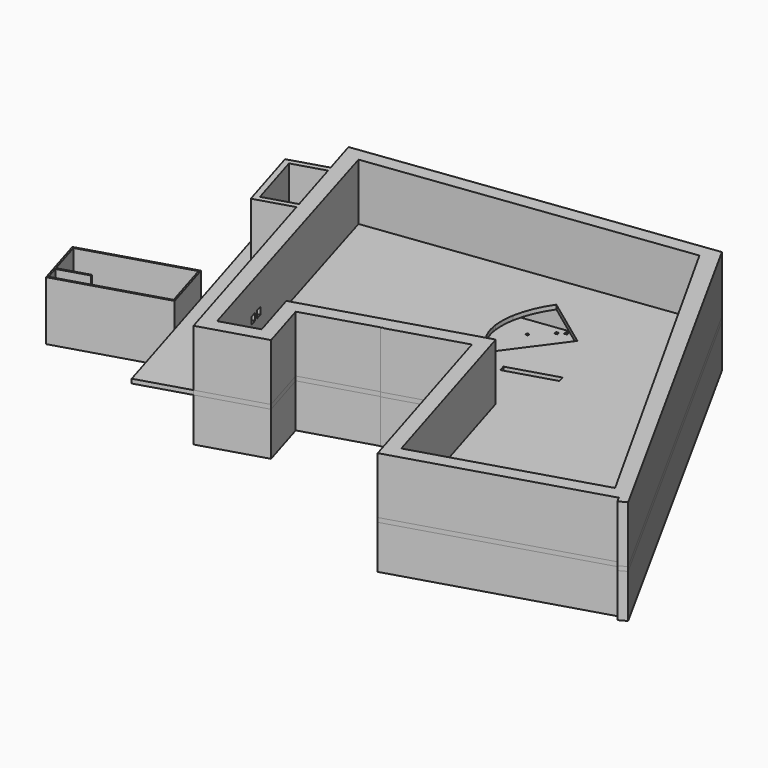
from build123d import *

# Parameters (mm, degrees)
F1_R      = 75
F1_R_2    = 100
F1_R_3    = 150
F1_R_4    = 50
F2_DEPTH  = 400
F4_DEPTH  = 2680
F7_DEPTH  = 2680
F9_DEPTH  = 300
F11_DEPTH = 4000
F14_DEPTH = 1900
F12_W     = 500
F12_H     = 500
F15_DEPTH = 16915.5989171206
F18_DEPTH = 63
F20_DEPTH = 910
F22_DEPTH = 2156
F24_DEPTH = 1900
F27_DEPTH = 2680
F29_DEPTH = 3760


# Not quite as in the source:
# - ends of sketch curves that miss each other by under 0.0002 mm in the source are joined
# - a feature names something its author has since deleted; it is built from what else it names


with BuildPart() as f2:
    # F1 (on Top) → F2 (new body)
    with BuildSketch(Plane.XY):
        Polygon((68188.427711, 49622.941476), (53564.501612, 76178.386836), (29657.706749, 73111.614693), (36317.523535, 51108.764438), (40724.124581, 52442.553255), (39664.460875, 55943.493684), (44744.962242, 57481.258468), (44495.221452, 57370.0585), (49699.0721480633, 58945.1162273297), (53744.872467, 45578.511492), (67446.814258, 49725.811541), (67662.852275, 49333.510204), align=None)
        Polygon((36888.614693, 52850.018992), (37127.489516, 52922.321559), (37272.339547, 52443.762818), (37033.464724, 52371.460251), align=None, mode=Mode.SUBTRACT)
        Polygon((38337.688965, 53575.367629), (37715.562601, 53387.062589), (37367.922527, 54535.603567), (37990.048891, 54723.908607), align=None, mode=Mode.SUBTRACT)
        with Locations((35374.891145, 58281.843639)):
            Circle(F1_R, mode=Mode.SUBTRACT)
        with Locations((35316.951132, 58473.267135)):
            Circle(F1_R, mode=Mode.SUBTRACT)
        with Locations((34859.774665, 59971.761029)):
            Circle(F1_R_2, mode=Mode.SUBTRACT)
        Polygon((34666.295724, 60274.624132), (34857.719221, 60332.564144), (34915.659233, 60141.140648), (34724.235737, 60083.200636), align=None, mode=Mode.SUBTRACT)
        with BuildLine():
            ThreePointArc((34784.617120491, 60519.2635586864), (34807.8959168534, 60486.099361855), (34816.1047484112, 60446.4208866322))
            ThreePointArc((34816.1047484112, 60446.4208866322), (34704.5717317165, 60347.0881653067), (34618.7649578928, 60469.3330052997))
            ThreePointArc((34618.7649578928, 60469.3330052997), (34591.5225392509, 60513.3482589154), (34589.9375394542, 60565.0877960215))
            ThreePointArc((34589.9375394542, 60565.0877960215), (34562.6951208123, 60609.1030496371), (34561.1101210156, 60660.8425867432))
            ThreePointArc((34561.1101210156, 60660.8425867432), (34589.9440178726, 60825.4764272397), (34729.6224930954, 60733.6852587974))
            ThreePointArc((34729.6224930954, 60733.6852587974), (34728.9552144209, 60722.1522421027), (34726.9622836138, 60710.7731401299))
            ThreePointArc((34726.9622836138, 60710.7731401299), (34750.2410799763, 60677.6089432985), (34758.449911534, 60637.9304680757))
            ThreePointArc((34758.449911534, 60637.9304680757), (34757.7826328595, 60626.397451381), (34755.7897020524, 60615.0183494082))
            ThreePointArc((34755.7897020524, 60615.0183494082), (34779.0684984148, 60581.8541525768), (34787.2773299726, 60542.1756773539))
            ThreePointArc((34787.2773299726, 60542.1756773539), (34786.6100512981, 60530.6426606592), (34784.617120491, 60519.2635586864))
        make_face(mode=Mode.SUBTRACT)
        Polygon((39127.684725, 56827.0438), (38801.772155, 57903.800968), (42989.161139, 59171.238737), (43315.073708, 58094.48157), align=None, mode=Mode.SUBTRACT)
        with BuildLine():
            ThreePointArc((60275.4999196738, 49676.0403187225), (60314.105205872, 49648.9704490009), (60328.926179, 49604.210146))
            ThreePointArc((60328.926179, 49604.210146), (60228.5191784936, 49533.6446847228), (60196.1399303262, 49652.0196582775))
            ThreePointArc((60196.1399303262, 49652.0196582775), (60172.9533679991, 49784.028857872), (60292.713671, 49723.849831))
            ThreePointArc((60292.713671, 49723.849831), (60288.2791322772, 49698.4428304936), (60275.4999196738, 49676.0403187225))
        make_face(mode=Mode.SUBTRACT)
        with Locations((60065.621139, 50226.336509)):
            Circle(F1_R_2, mode=Mode.SUBTRACT)
        with Locations((60145.288655, 49963.129201)):
            Circle(F1_R, mode=Mode.SUBTRACT)
        Polygon((32914.905569, 66064.012816), (33106.329065, 66121.952828), (33164.269078, 65930.529332), (32972.845581, 65872.58932), align=None, mode=Mode.SUBTRACT)
        with Locations((33845.60075, 63524.719235)):
            Circle(F1_R_3, mode=Mode.SUBTRACT)
        with Locations((39975.073073, 63798.527996)):
            Circle(F1_R_2, mode=Mode.SUBTRACT)
        with Locations((42925.067085, 63312.529711)):
            Circle(F1_R_2, mode=Mode.SUBTRACT)
        with Locations((43205.184131, 63546.230085)):
            Circle(F1_R, mode=Mode.SUBTRACT)
        with Locations((42403.039755, 66446.164261)):
            Circle(F1_R_2, mode=Mode.SUBTRACT)
        with Locations((44009.013922, 66971.090202)):
            Circle(F1_R_4, mode=Mode.SUBTRACT)
        Polygon((41996.362564, 67627.28381), (42114.914654, 67788.359575), (42275.990419, 67669.807485), (42157.438329, 67508.73172), align=None, mode=Mode.SUBTRACT)
        Polygon((33353.336387, 67923.500203), (32032.970739, 72408.167064), (39441.151163, 73358.444069), (40436.811419, 70067.58033), align=None, mode=Mode.SUBTRACT)
        Polygon((41945.236424, 69090.172465), (42136.659921, 69148.112478), (42194.599933, 68956.688981), (42003.176437, 68898.748969), align=None, mode=Mode.SUBTRACT)
        with Locations((42962.383909, 72270.769883)):
            Circle(F1_R_2, mode=Mode.SUBTRACT)
        Polygon((44039.799467, 73281.109422), (44014.36577, 73479.485648), (44212.741996, 73504.919344), (44238.175693, 73306.543118), align=None, mode=Mode.SUBTRACT)
        Polygon((44450.636875, 73788.993839), (44649.013101, 73814.427535), (44674.446797, 73616.051309), (44476.070571, 73590.617613), align=None, mode=Mode.SUBTRACT)
        Polygon((51272.914035, 64941.22135), (51403.266417, 64510.514656), (48119.062842, 63518.921773), (48056.219999, 63967.696362), align=None, mode=Mode.SUBTRACT)
        Polygon((51543.488161, 65785.533894), (51615.907166, 65546.252705), (50850.207359, 65314.511888), (50777.788354, 65553.793078), align=None, mode=Mode.SUBTRACT)
        with Locations((46278.12246, 72377.01959)):
            Circle(F1_R, mode=Mode.SUBTRACT)
        with Locations((46019.965632, 73321.406391)):
            Circle(F1_R_4, mode=Mode.SUBTRACT)
        Polygon((47517.023596, 74394.419855), (48012.959721, 74458.038718), (48044.715372, 74210.489893), (47548.779247, 74146.87103), align=None, mode=Mode.SUBTRACT)
        Polygon((49750.603625, 74680.655926), (50345.773903, 74756.631841), (50421.749818, 74161.461563), (49826.579539, 74085.485648), align=None, mode=Mode.SUBTRACT)
        with Locations((51206.187105, 74656.133134)):
            Circle(F1_R, mode=Mode.SUBTRACT)
        with Locations((51528.343707, 74753.643407)):
            Circle(F1_R, mode=Mode.SUBTRACT)
    extrude(amount=F2_DEPTH)

    # F3 (on face) → F4 (join)
    with BuildSketch(Plane.XY.offset(400)):
        Polygon((29657.706749, 73111.614693), (36317.523535, 51108.764438), (40724.124581, 52442.553255), (39664.460875, 55943.493684), (44744.962242, 57481.258468), (44495.221452, 57370.0585), (49699.0721480633, 58945.1162273297), (53744.872467, 45578.511492), (67446.814258, 49725.811541), (67662.852275, 49333.510204), (68188.427711, 49622.941476), (53564.501612, 76178.386836), align=None)
        Polygon((38457.331895, 56624.200376), (39517.019236, 53123.181861), (36984.578302, 52356.663322), (32877.8040575006, 66091.2951018729), (31027.582141, 72279.148444), (52857.629236, 75079.514645), (66562.2744, 50502.75788), (54412.257067, 46825.252699), (50354.925373, 60229.993775), align=None, mode=Mode.SUBTRACT)
    extrude(amount=F4_DEPTH)

    # F6 (on face) → F7 (join)
    with BuildSketch(Plane.XY.offset(400)):
        Polygon((41369.595174, 67281.80667), (41611.208821, 67103.978536), (42174.331247, 67869.088419), (41932.717599, 68046.916553), align=None)
        Polygon((39375.141872, 64572.389618), (38841.657469, 63847.548675), (39083.271116, 63669.720541), (39616.755519, 64394.561483), align=None)
        Polygon((35364.5019, 67249.581852), (34646.670423, 67032.26192), (34733.597625, 66745.131877), (35451.429101, 66962.451809), align=None)
        Polygon((52648.50255, 73503.687457), (52380.653898, 73984.059291), (52162.303064, 73862.309903), (52430.151717, 73381.938069), align=None)
        Polygon((49677.774159, 74066.592025), (49601.798244, 74661.762303), (49304.213105, 74623.774346), (49380.18902, 74028.604068), align=None)
        Polygon((49895.571781, 72360.437227), (49697.181689, 72335.111922), (49814.944357, 71412.59799), (50013.334449, 71437.923295), align=None)
        Polygon((51120.461189, 69456.928766), (50876.962414, 69893.630434), (50444.203241, 69652.329938), (50687.702016, 69215.628271), align=None)
        Polygon((53406.432689, 64339.734264), (53838.911214, 64580.878274), (53595.412439, 65017.579941), (53162.933913, 64776.435931), align=None)
        Polygon((56309.873132, 59132.573438), (56736.195141, 59370.284661), (56492.696366, 59806.986328), (56066.374356, 59569.275106), align=None)
        Polygon((58655.376546, 54926.042001), (59081.698556, 55163.753223), (58838.199781, 55600.454891), (58411.877771, 55362.743669), align=None)
        Polygon((61456.104007, 50905.387575), (61212.605232, 51342.089242), (60786.283222, 51104.37802), (61029.781997, 50667.676352), align=None)
    extrude(amount=F7_DEPTH)

    # F26 (on face) → F27 (join)
    with BuildSketch(Plane.XY.offset(400)):
        Polygon((37619.064125, 61069.110952), (37824.844383, 61131.396467), (37790.7700244054, 61243.97208482), (41542.214678, 62379.458373), (41576.289045, 62266.882727), (41782.069304, 62329.168242), (41747.994936, 62441.743888), (41963.434855, 62506.953186), (41901.14934, 62712.733444), (37728.484511, 61449.752343), (36836.955295, 64395.206235), (40930.85491, 69983.095387), (41638.0882945605, 67646.606100707), (41797.2602227136, 67862.8717117348), (40107.9121949509, 73443.976410992), (39891.6750244535, 73416.2374298975), (40852.932564, 70240.527699), (36600.074516, 64435.671306), align=None)
        Polygon((38921.8380103628, 56764.9778439533), (38924.037933, 56757.709691), (39129.818191, 56819.995206), (38801.7721485487, 57903.8009595607), (42758.997061, 59101.572763), (42045.696378, 61458.191297), (41839.91612, 61395.905783), (41889.8547615391, 61230.9173971632), (40476.084233, 60802.997703), (40538.369747, 60597.217445), (41952.140276, 61025.137139), (42490.931288, 59245.067506), (38739.486635, 58109.581218), (38200.6956220125, 59889.6508510038), (39667.392841, 60333.590382), (39605.107326, 60539.37064), (38138.410107, 60095.431109), (38088.471446, 60260.41956), (37882.691188, 60198.134046), align=None)
        Polygon((43824.9103409903, 60275.5110113383), (43861.137757, 60155.859535), (44385.9222448319, 58422.6076047011), (44672.8132943379, 58509.3286146567), (44184.431224, 60123.127126), (44643.845234, 60262.17825), (44571.422215, 60501.458225), (44111.0388549428, 60362.113706791), (43745.9906283531, 61568.1681271069), (43745.9834585876, 61568.1918134635), (43648.270567, 61891.017829), (43442.490309, 61828.732315), (43540.2086068099, 61505.8884359628), (43459.758486, 61481.530191), align=None)
        Polygon((46634.171938, 61125.317628), (45433.204423, 60761.820044), (45432.961644444, 60761.7465620636), (45469.041634, 60642.541104), (45505.253143, 60522.901117), (45964.6971664966, 60661.9613250455), (46453.3185102622, 59047.5371465089), (46644.721342085, 59105.5454377498), (46156.121537, 60719.89845), (46706.463437, 60886.472183), align=None)
        Polygon((43282.95358, 63097.960184), (44828.639678, 65198.312762), (41831.816909, 67403.72691), (41704.382914, 67230.563471), (44528.042243, 65152.583318), (42970.76907, 63036.485665), (42772.126247, 62976.360507), (42834.411762, 62770.580249), (43130.303868, 62860.140795), (43149.893247, 62795.420972), (43355.673505, 62857.706486), align=None)
        Polygon((47759.295327, 61205.133465), (48505.850149, 61431.093677), (48994.2066954253, 59817.6019384015), (49233.460234103, 59890.1123021189), (48672.707105, 61742.796671), (47686.872308, 61444.41344), (47723.083817, 61324.773453), align=None)
    extrude(amount=F27_DEPTH)


with BuildPart() as f2b:
    # F1 (on Top) → F2, piece 2 (new body)
    with BuildSketch(Plane.XY):
        Polygon((29791.9764274075, 57600.7037435227), (28663.3049876725, 61329.6334533894), (21355.7130126129, 59117.7734835802), (22484.3844523479, 55388.8437737135), align=None)
    extrude(amount=F2_DEPTH)

    # F28 (on face) → F29 (join)
    with BuildSketch(Plane.XY.offset(400)):
        Polygon((29791.9764274075, 57600.7037435227), (28663.3049876725, 61329.6334533894), (21355.7130126129, 59117.7734835802), (22484.3844523479, 55388.8437737135), align=None)
        Polygon((28591.777658216, 61203.5031987285), (29661.0605853366, 57670.7825726715), (22554.4632814967, 55519.7596157844), (22264.7632199631, 56476.877097783), (24307.5083095779, 57095.1746310421), (24278.5383034245, 57190.886379242), (22235.7932138097, 56572.5888459829), (21485.1803543761, 59052.4802418414), align=None, mode=Mode.SUBTRACT)
    extrude(amount=F29_DEPTH)


with BuildPart() as f9:
    # F8 (on face) → F9 (new body)
    with BuildSketch(Plane.XY.offset(3080)):
        Polygon((68188.427711, 49622.941476), (53564.501612, 76178.386836), (29657.706749, 73111.614693), (26143.6735266067, 72047.9880641845), (32803.4903126067, 50045.1378091846), (36317.523535, 51108.764438), (40724.124581, 52442.553255), (39664.460875, 55943.493684), (44744.962242, 57481.258468), (44495.221452, 57370.0585), (49699.0721480633, 58945.1162273297), (53744.872467, 45578.511492), (67446.814258, 49725.811541), (67662.852275, 49333.510204), align=None)
        Polygon((35054.3479230535, 58812.0957190118), (35463.9358685144, 58934.5660736769), (38413.86064, 56763.63706), (38457.331895, 56624.200376), (39517.019236, 53123.181861), (36984.578302, 52356.663322), align=None, mode=Mode.SUBTRACT)
        with BuildLine():
            Line((45559.414096, 71574.528756), (49171.713743, 68915.43602))
            Line((49171.713743, 68915.43602), (46261.512692, 64962.013078))
            ThreePointArc((46261.512692, 64962.013078), (45571.8751044626, 65400.6858874001), (45027.1641833529, 66010.0493652373))
            ThreePointArc((45027.1641833529, 66010.0493652373), (44899.5564047433, 66220.6886656855), (44786.6520625048, 66439.5613902401))
            ThreePointArc((44786.6520625048, 66439.5613902401), (44617.0942694773, 66866.3247002513), (44503.2553788585, 67311.2038691621))
            ThreePointArc((44503.2553788585, 67311.2038691621), (44497.2447415665, 67345.187388798), (44491.4738453053, 67379.2124402223))
            ThreePointArc((44491.4738453053, 67379.2124402223), (44475.4844701719, 67479.9554221894), (44462.2724974932, 67581.1001319409))
            ThreePointArc((44462.2724974932, 67581.1001319409), (44427.3713892882, 68319.4085470206), (44504.0329082882, 69054.5550729477))
            ThreePointArc((44504.0329082882, 69054.5550729477), (44896.7275643795, 70371.0790815159), (45559.414096, 71574.528756))
        make_face(mode=Mode.SUBTRACT)
        Polygon((51388.2570420098, 64560.1107619676), (48028.730664, 63543.315669), (47898.373323, 63974.020862), (51257.8997, 64990.815955), align=None, mode=Mode.SUBTRACT)
    extrude(amount=F9_DEPTH)


with BuildPart() as f11:
    # F10 (on face) → F11 (new body)
    with BuildSketch(Plane.XY.offset(3380)):
        Polygon((31896.3185086878, 65715.6395618169), (36317.523535, 51108.764438), (40724.124581, 52442.553255), (39664.460875, 55943.493684), (44744.962242, 57481.258468), (44495.221452, 57370.0585), (49699.0721480633, 58945.1162273297), (53744.872467, 45578.511492), (67446.814258, 49725.811541), (67662.852275, 49333.510204), (68188.427711, 49622.941476), (53564.501612, 76178.386836), (29657.706749, 73111.614693), (30424.9273433281, 70576.8542946301), (27830.2423117378, 69791.4957283613), (29301.6334772496, 64930.2809956998), align=None)
        Polygon((29561.9272038867, 65416.5415800144), (28316.5028960663, 69531.2020017285), (30537.9107721759, 70203.5771391494), (31783.3350798539, 66088.9167173017), align=None, mode=Mode.SUBTRACT)
        Polygon((38457.331895, 56624.200376), (39517.019236, 53123.181861), (36984.578302, 52356.663322), (32877.8040575006, 66091.2951018729), (31027.582141, 72279.148444), (52857.629236, 75079.514645), (66562.2744, 50502.75788), (54412.257067, 46825.252699), (50354.925373, 60229.993775), align=None, mode=Mode.SUBTRACT)
    extrude(amount=F11_DEPTH)

    # F12 (on face) → F15 (cut, through all)
    with BuildSketch(Plane(origin=(48319.6036101898, 14447.981335877, 0), x_dir=(-0.2864764251, 0.9580872914, 0), z_dir=(0.9580872914, 0.2864764251, 0))):
        with Locations((45686.4227301382, 4955)):
            Rectangle(F12_W, F12_H)
        with Locations((44886.4227301382, 4955)):
            Rectangle(F12_W, F12_H)
    extrude(amount=-F15_DEPTH, mode=Mode.SUBTRACT)


with BuildPart() as f14:
    # F13 (on Top) → F14 (new body)
    with BuildSketch(Plane.XY):
        Polygon((37404.4760965891, 56508.7168304175), (36671.5393186966, 56289.5623652278), (37026.7700858015, 55101.534123938), (37759.706863694, 55320.6885891277), align=None)
    extrude(amount=F14_DEPTH)


with BuildPart() as f18:
    # F17 (on face) → F18 (new body)
    with BuildSketch(Plane.XY.offset(400)):
        Polygon((34033.2469225817, 63972.3943066302), (34293.9419465539, 63100.5299313487), (34871.1444677788, 63275.2374349344), (34607.5174117803, 64146.2143435523), align=None)
    extrude(amount=F18_DEPTH)

    # F19 (on face) → F20 (join)
    with BuildSketch(Plane(origin=(-14618.1675423812, 48295.8258115735, 0), x_dir=(0.957117482, 0.2897000615, 0), z_dir=(0.2897000615, -0.957117482, 0))):
        with BuildLine():
            Line((51706.6221660345, 463), (51647.3741336438, 542.9715229036))
            ThreePointArc((51647.3741336438, 542.9715229035), (51405.0904669059, 1277), (51162.806800168, 542.9715229036))
            Line((51162.806800168, 542.9715229036), (51103.5587677773, 463))
            Line((51103.5587677773, 463), (51706.6221660345, 463))
        make_face()
        with BuildLine():
            ThreePointArc((51446.2912820725, 548.8655742304), (51345.0387756051, 551.8512596966), (51249.664547087, 585.9795605362))
            Line((51249.664547087, 585.9795605362), (51348.6656883736, 766.8911336406))
            ThreePointArc((51348.6656883736, 766.8911336406), (51383.289705578, 754.5014252908), (51420.0477331961, 753.4175221594))
            Line((51420.0477331961, 753.4175221594), (51446.2912820725, 548.8655742304))
        make_face(mode=Mode.SUBTRACT)
        with BuildLine():
            Line((51086.9417266025, 930.0516913007), (51289.5918921967, 891.8007613279))
            ThreePointArc((51289.5918921967, 891.8007613279), (51288.5079890653, 855.0427337098), (51298.8359911428, 819.7488275297))
            Line((51298.8359911428, 819.7488275297), (51112.4052307396, 731.5797012175))
            ThreePointArc((51112.4052307396, 731.5797012175), (51083.9560411363, 828.7991848334), (51086.9417266025, 930.0516913007))
        make_face(mode=Mode.SUBTRACT)
        with BuildLine():
            Line((51627.1807060286, 634.414023611), (51485.7166106745, 784.4744547206))
            ThreePointArc((51485.7166106745, 784.4744547206), (51508.1993332653, 813.5752214677), (51520.5890416151, 848.1992386721))
            Line((51520.5890416151, 848.1992386721), (51723.2392072093, 809.9483086993))
            ThreePointArc((51723.2392072093, 809.9483086993), (51689.1109063697, 714.5740801811), (51627.1807060286, 634.414023611))
        make_face(mode=Mode.SUBTRACT)
        with BuildLine():
            Line((51363.8896517392, 1191.1344257696), (51390.1332006157, 986.5824778406))
            ThreePointArc((51390.1332006157, 986.5824778406), (51354.8392944355, 976.2544757631), (51324.4643231373, 955.5255452794))
            Line((51324.4643231373, 955.5255452794), (51183.0002277832, 1105.585976389))
            ThreePointArc((51183.0002277832, 1105.585976389), (51266.6701681234, 1162.6852361663), (51363.8896517393, 1191.1344257696))
        make_face(mode=Mode.SUBTRACT)
        with BuildLine():
            Line((51697.7757030721, 1008.4202987825), (51511.344942669, 920.2511724703))
            ThreePointArc((51511.344942669, 920.2511724703), (51490.6160121853, 950.6261437686), (51461.5152454382, 973.1088663594))
            Line((51461.5152454382, 973.1088663594), (51560.5163867247, 1154.0204394638))
            ThreePointArc((51560.5163867247, 1154.0204394638), (51640.6764432949, 1092.0902391227), (51697.7757030721, 1008.4202987825))
        make_face(mode=Mode.SUBTRACT)
    extrude(amount=-F20_DEPTH)


with BuildPart() as f22:
    # F21 (on face) → F22 (new body)
    with BuildSketch(Plane.XY.offset(400)):
        Polygon((36487.7295639419, 68872.242182117), (35243.479555764, 68495.6231210626), (36170.5418598978, 65432.8538701634), (37414.7918680756, 65809.4729312177), align=None)
    extrude(amount=F22_DEPTH)


with BuildPart() as f24:
    # F23 (on face) → F24 (new body)
    with BuildSketch(Plane.XY.offset(400)):
        Polygon((37239.5926870895, 59560.4500847429), (36970.1716298497, 60450.5693429975), (36237.9767561241, 60228.9487959131), (36507.397813364, 59338.8295376585), align=None)
    extrude(amount=F24_DEPTH)


solid = Compound([f2.part, f2b.part, f9.part, f11.part, f14.part, f18.part, f22.part, f24.part])
